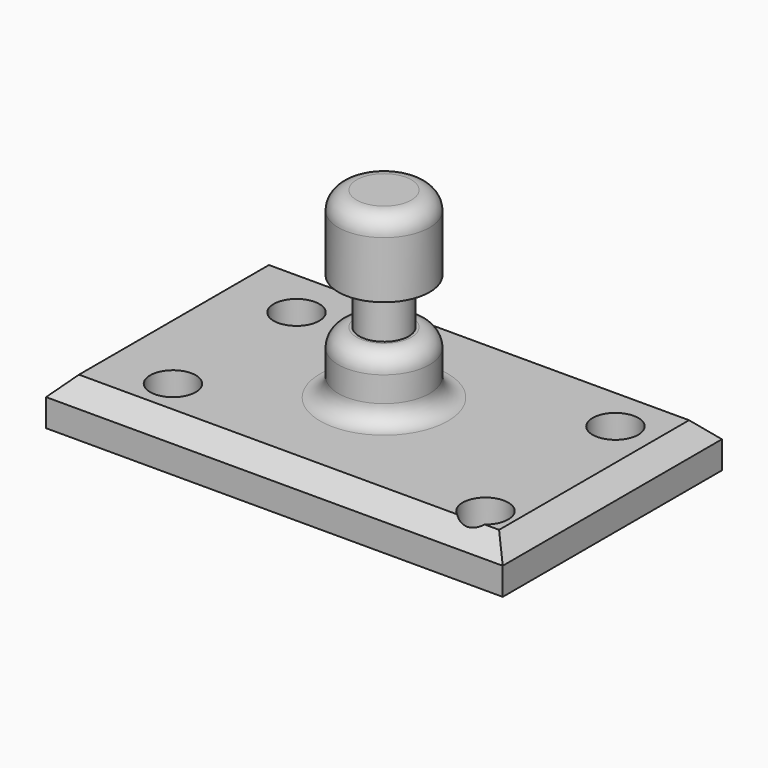
from build123d import *

# Parameters (mm, degrees)
F0_W        = 127
F0_H        = 76.2
F1_DEPTH    = 12.7
F2_R        = 6.35
F3_DEPTH    = 12.701
F4_W        = 12.7
F4_H        = 50.8
F6_W        = 7.62
F6_H        = 12.7
F8_R        = 5.08
F9_T1_DEPTH = 153.1282991577
F9_T3_DEPTH = 102.3282991577


# Not quite as in the source:
# - a fillet or chamfer that OpenCascade refuses, or shapes differently, is made with other operations: its cross-section is extruded or revolved along the edge and cut away or added


with BuildPart() as f1:
    # F0 (on Top) → F1 (new body)
    with BuildSketch(Plane.XY):
        Rectangle(F0_W, F0_H)
    extrude(amount=F1_DEPTH)

    # F2 (on face) → F3 (cut, through all)
    with BuildSketch(Plane.XY.offset(12.7)):
        with Locations((-39.8141870437, -23.5891287784)):
            Circle(F2_R)
        with Locations((47.751432499, 20.7712577737)):
            Circle(F2_R)
        with Locations((-39.8141870437, 19.3517001108)):
            Circle(F2_R)
        with Locations((50.5741164088, -27.9485974461)):
            Circle(F2_R)
    extrude(amount=-F3_DEPTH, mode=Mode.SUBTRACT)

    # F4 (on Front) → F5 (revolve)
    with BuildSketch(Plane.XZ):
        with Locations((6.35, 38.1)):
            Rectangle(F4_W, F4_H)
    revolve(axis=Axis((0, 0, 38.1), (0, 0, 1)))

    # F6 (on Front) → F7 (revolve, cut)
    with BuildSketch(Plane.XZ):
        with Locations((10.6961938009, 36.2604726106)):
            Rectangle(F6_W, F6_H)
    revolve(axis=Axis((0, 0, 12.7), (0, 0, 1)), mode=Mode.SUBTRACT)

    # F8
    f8_edges = [f1.edges().sort_by_distance(p)[0] for p in [
        (-12.7, 0, 29.910473),
        (-12.7, 0, 63.5),
        (-12.7, 0, 12.7),
    ]]
    fillet(f8_edges, radius=F8_R)

    # F9: chamfer of 5.08 on 7 edges, made by hand

    # F9_s2 → F9_t1 (cut)
    with BuildSketch(Plane.YZ.offset(-76.5641495789)):
        Polygon((33.02, 12.7), (38.1, 7.62), (38.1, 12.7), align=None)
        Polygon((-33.02, 12.7), (-38.1, 7.62), (-38.1, 12.7), align=None)
    extrude(amount=F9_T1_DEPTH, mode=Mode.SUBTRACT)

    # F9_s4 → F9_t3 (cut)
    with BuildSketch(Plane.XZ.offset(-51.1641495789)):
        Polygon((58.42, 12.7), (63.5, 7.62), (63.5, 12.7), align=None)
        Polygon((-58.42, 12.7), (-63.5, 7.62), (-63.5, 12.7), align=None)
    extrude(amount=F9_T3_DEPTH, mode=Mode.SUBTRACT)


solid = f1.part
